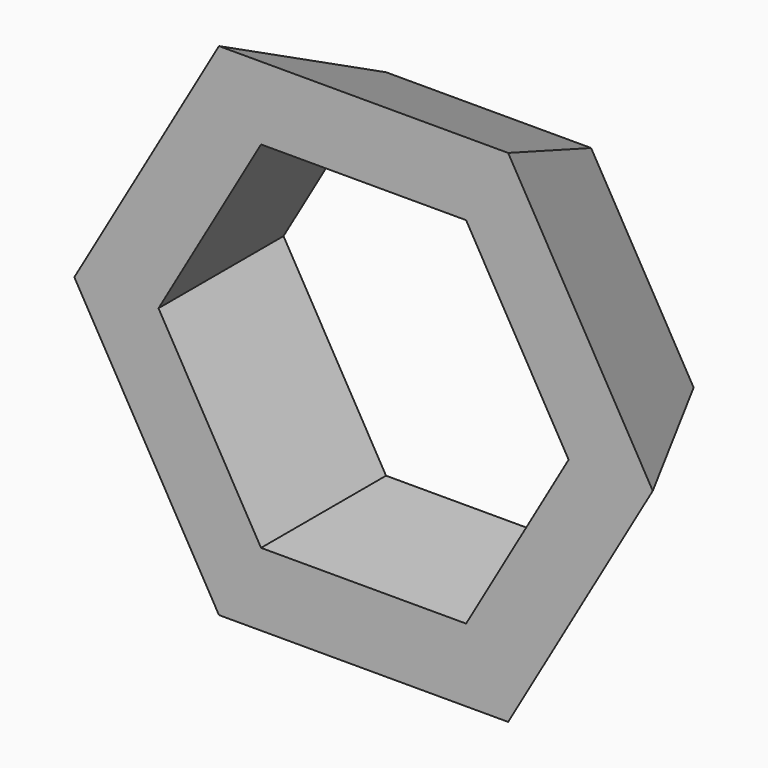
from build123d import *

# Parameters (mm, degrees)
F1_DEPTH    = 25.4
F2_T1_DEPTH = 176.9830394525
F2_T3_DEPTH = 176.9830394525
F2_T5_DEPTH = 176.9830394525
F2_T7_DEPTH = 176.9830394525
F2_T9_DEPTH = 176.9830394525


# Not quite as in the source:
# - a fillet or chamfer that OpenCascade refuses, or shapes differently, is made with other operations: its cross-section is extruded or revolved along the edge and cut away or added


with BuildPart() as f1:
    # F0 (on Front) → F1 (new body)
    with BuildSketch(Plane.XZ):
        Polygon((7.0658522586, 57.8397729191), (-38.2956332455, 57.8397729191), (-60.9763759976, 18.5555741191), (-38.2956332455, -20.7286246809), (7.0658522586, -20.7286246809), (29.7465950107, 18.5555741191), align=None)
        Polygon((16.548367857, 18.5555741191), (0.4667386818, -9.2986246809), (-31.6965196687, -9.2986246809), (-47.7781488439, 18.5555741191), (-31.6965196687, 46.4097729191), (0.4667386818, 46.4097729191), align=None, mode=Mode.SUBTRACT)
    extrude(amount=-F1_DEPTH)

    # F2: chamfer of 25.4 x 11.8442145171 on 6 edges, made by hand

    # F2_s2 → F2_t1 (cut)
    with BuildSketch(Plane.YZ.offset(-104.1064102197)):
        Polygon((0, 57.8397729191), (25.4, 45.995558402), (25.4, 57.8397729191), align=None)
        Polygon((0, -20.7286246809), (25.4, -8.8844101638), (25.4, -20.7286246809), align=None)
    extrude(amount=F2_T1_DEPTH, mode=Mode.SUBTRACT)

    # F2_s4 → F2_t3 (cut)
    with BuildSketch(Plane(origin=(48.3768365242, 0, 83.7911387694), x_dir=(0, 1, 0), z_dir=(-0.5, 0, -0.8660254038))):
        Polygon((0, -62.0848777042), (25.4, -50.2406631871), (25.4, -62.0848777042), align=None)
    extrude(amount=F2_T3_DEPTH, mode=Mode.SUBTRACT)

    # F2_s6 → F2_t5 (cut)
    with BuildSketch(Plane(origin=(32.3072379553, 0, -55.9577775908), x_dir=(0, 1, 0), z_dir=(-0.5, 0, 0.8660254038))):
        Polygon((0, -35.0390940149), (25.4, -23.1948794978), (25.4, -35.0390940149), align=None)
    extrude(amount=F2_T5_DEPTH, mode=Mode.SUBTRACT)

    # F2_s8 → F2_t7 (cut)
    with BuildSketch(Plane(origin=(-40.114683202, 0, -69.4806694354), x_dir=(0, 1, 0), z_dir=(0.5, 0, 0.8660254038))):
        Polygon((0, -16.4835198958), (25.4, -4.6393053787), (25.4, -16.4835198958), align=None)
    extrude(amount=F2_T7_DEPTH, mode=Mode.SUBTRACT)

    # F2_s10 → F2_t9 (cut)
    with BuildSketch(Plane(origin=(-56.184281771, 0, 97.3140306141), x_dir=(0, 1, 0), z_dir=(0.5, 0, -0.8660254038))):
        Polygon((0, -43.5293035851), (25.4, -31.685089068), (25.4, -43.5293035851), align=None)
    extrude(amount=F2_T9_DEPTH, mode=Mode.SUBTRACT)


solid = f1.part
